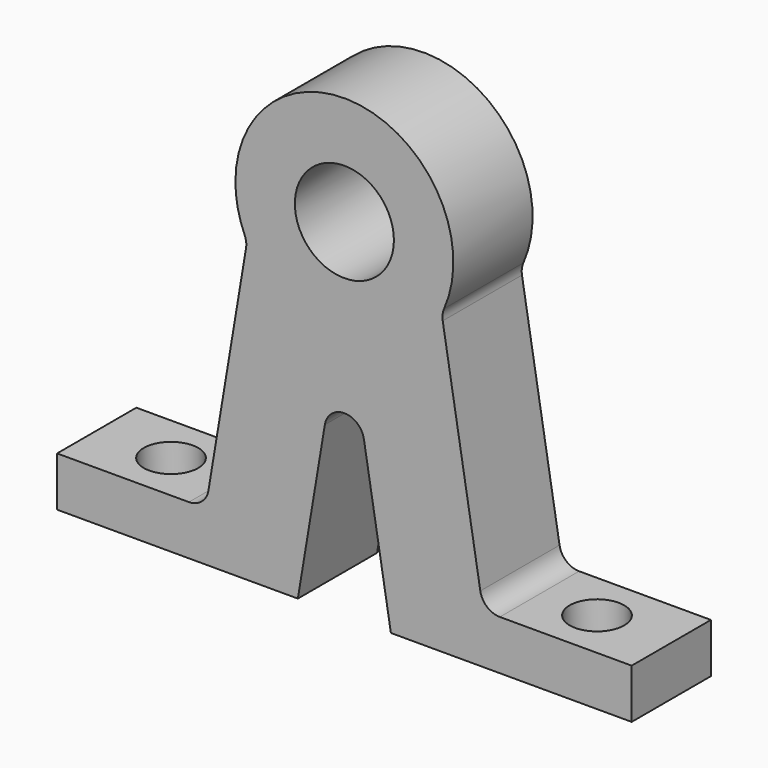
from build123d import *

# Parameters (mm, degrees)
F0_R     = 5
F1_DEPTH = 10
F2_R     = 2.75
F3_DEPTH = 5.001
F4_R     = 5
F5_DEPTH = 10
F6_R     = 2


with BuildPart() as f1:
    # F0 (on Front) → F1 (new body)
    with BuildSketch(Plane.XZ):
        with BuildLine():
            ThreePointArc((-0.3608562494, -8.9927627995), (-6.4902891401, -6.2350739272), (-9, 0))
            Line((-9, 0), (-14, -30))
            Line((-14, -30), (-29, -30))
            Line((-29, -30), (-29, -35))
            Line((-29, -35), (-4.6953957828, -35))
            Line((-4.6953957828, -35), (-0.3608562494, -8.9927627995))
        make_face()
        with BuildLine():
            ThreePointArc((0.3608562494, -8.9927627995), (6.4902891401, -6.2350739272), (9, 0))
            ThreePointArc((9, 0), (0, 9), (-9, 0))
            ThreePointArc((-9, 0), (-6.4902891401, -6.2350739272), (-0.3608562494, -8.9927627995))
            Line((-0.3608562494, -8.9927627995), (0, -6.827625303))
            Line((0, -6.827625303), (0.3608562494, -8.9927627995))
        make_face()
        Circle(F0_R, mode=Mode.SUBTRACT)
        with BuildLine():
            Line((14, -30), (9, 0))
            ThreePointArc((9, 0), (6.4902891401, -6.2350739272), (0.3608562494, -8.9927627995))
            Line((0.3608562494, -8.9927627995), (4.6953957828, -35))
            Line((4.6953957828, -35), (29, -35))
            Line((29, -35), (29, -30))
            Line((29, -30), (14, -30))
        make_face()
    extrude(amount=F1_DEPTH)

    # F2 (on face) → F3 (cut, through all)
    with BuildSketch(Plane.XY.offset(-30)):
        with Locations((-21.5, -5)):
            Circle(F2_R)
        with Locations((21.5, -5)):
            Circle(F2_R)
    extrude(amount=-F3_DEPTH, mode=Mode.SUBTRACT)

    # F4 (on face) → F5 (join, through all)
    with BuildSketch(Plane(origin=(0, 0, 0), x_dir=(-1, 0, 0), z_dir=(0, 1, 0))):
        with BuildLine():
            ThreePointArc((9.8245808792, -4.9474852752), (10.7021116998, -2.542598113), (11, 0))
            ThreePointArc((11, 0), (-2.542598113, 10.7021116998), (-9.8245808792, -4.9474852752))
            Line((-9.8245808792, -4.9474852752), (-9, 0))
            ThreePointArc((-9, 0), (0, 9), (9, 0))
            Line((9, 0), (9.8245808792, -4.9474852752))
        make_face()
        with BuildLine():
            Line((-9, 0), (-9.8245808792, -4.9474852752))
            ThreePointArc((-9.8245808792, -4.9474852752), (-6.0614233206, -9.1792781485), (-0.6917668776, -10.9782265684))
            Line((-0.6917668776, -10.9782265684), (0, -6.827625303))
            Line((0, -6.827625303), (0.6917668776, -10.9782265684))
            ThreePointArc((0.6917668776, -10.9782265684), (6.0614233206, -9.1792781485), (9.8245808792, -4.9474852752))
            Line((9.8245808792, -4.9474852752), (9, 0))
            ThreePointArc((9, 0), (0, 9), (-9, 0))
        make_face()
        Circle(F4_R, mode=Mode.SUBTRACT)
    extrude(amount=-F5_DEPTH)

    # F6
    f6_edges = [f1.edges().sort_by_distance(p)[0] for p in [
        (0, -5, -6.827625),
        (-14, -5, -30),
        (14, -5, -30),
        (-9.824581, -5, -4.947485),
        (9.824581, -5, -4.947485),
    ]]
    fillet(f6_edges, radius=F6_R)


solid = f1.part
